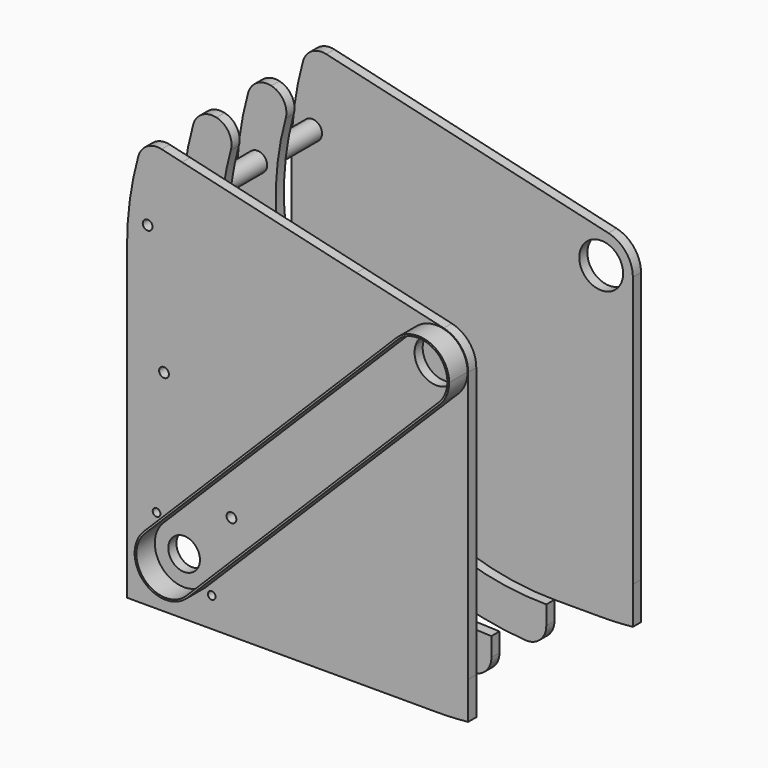
from build123d import *

# Parameters (mm, degrees)
F0_R      = 2.4892
F0_R_2    = 19.1008
F0_R_3    = 3.175
F0_R_4    = 10.31875
F1_DEPTH  = 6.604
F2_R      = 6.35
F2_R_2    = 3.175
F3_DEPTH  = 38.1
F4_R      = 6.35
F4_R_2    = 3.175
F5_DEPTH  = 6.604
F6_R      = 6.35
F6_R_2    = 3.175
F7_DEPTH  = 38.1
F8_R      = 2.15265
F8_R_2    = 6.35
F8_R_3    = 3.175
F9_DEPTH  = 6.604
F10_R     = 6.35
F10_R_2   = 3.175
F10_R_3   = 2.15265
F11_DEPTH = 38.1
F12_R     = 3.175
F12_R_2   = 25.4
F12_R_3   = 14.2875
F12_R_4   = 6.35
F13_DEPTH = 6.604
F14_R     = 12.69999
F16_DEPTH = 15


# Not quite as in the source:
# - a fillet or chamfer is up to 0.001 mm smaller than in the source, because OpenCascade refuses the exact size


with BuildPart() as f1:
    # F0 (on Front) → F1 (new body)
    with BuildSketch(Plane.XZ):
        with BuildLine():
            Line((20.6375, -174.9998249999), (20.6375, -58.3716647869))
            ThreePointArc((20.6375, -58.3716647869), (-43.598353039, -43.9584038442), (-58.5394188118, 20.1567383628))
            Line((-58.5394188118, 20.1567383628), (-166.6121920028, 57.3691784173))
            ThreePointArc((-166.6121920028, 57.3691784173), (-143.4573307784, -102.3271195832), (0, -176.2125))
            ThreePointArc((0, -176.2125), (10.3365490724, -175.9090700036), (20.6375, -174.9998249999))
        make_face()
        with BuildLine():
            ThreePointArc((-92.0202423383, -179.3875), (-172.0465507714, -105.1074903321), (-201.6125, 0))
            Line((-201.6125, 0), (-201.6125, -201.6125))
            Line((-201.6125, -201.6125), (0, -201.6125))
            ThreePointArc((0, -201.6125), (-47.3330635629, -195.9775018975), (-92.0202423383, -179.3875))
        make_face()
        with Locations((-146.444987879, -182.3660123632)):
            Circle(F0_R, mode=Mode.SUBTRACT)
        with Locations((-164.4055001211, -164.4055001211)):
            Circle(F0_R_2, mode=Mode.SUBTRACT)
        with Locations((-182.3660123632, -146.444987879)):
            Circle(F0_R, mode=Mode.SUBTRACT)
        with BuildLine():
            ThreePointArc((0, -176.2125), (-143.4573307784, -102.3271195832), (-166.6121920028, 57.3691784173))
            Line((-166.6121920028, 57.3691784173), (-190.628363823, 65.6386095405))
            ThreePointArc((-190.628363823, 65.6386095405), (-198.8475058399, 33.2756604366), (-201.6125, 0))
            ThreePointArc((-201.6125, 0), (-172.0465507714, -105.1074903321), (-92.0202423383, -179.3875))
            Line((-92.0202423383, -179.3875), (20.6358525902, -179.3875))
            Line((20.6358525902, -179.3875), (20.6358525902, -176.2125))
            Line((20.6358525902, -176.2125), (0, -176.2125))
        make_face()
        with Locations((-133.5813098009, -133.5813098009)):
            Circle(F0_R_3, mode=Mode.SUBTRACT)
        with Locations((-177.5196822242, -64.611880326)):
            Circle(F0_R_3, mode=Mode.SUBTRACT)
        with Locations((-188.1936309033, 16.4648092518)):
            Circle(F0_R_3, mode=Mode.SUBTRACT)
        with BuildLine():
            ThreePointArc((-58.5394188118, 20.1567383628), (-43.598353039, -43.9584038442), (20.6375, -58.3716647869))
            Line((20.6375, -58.3716647869), (20.6375, 0))
            ThreePointArc((20.6375, 0), (-3.4061699659, -20.3544691017), (-19.5131396039, 6.7189127876))
            Line((-19.5131396039, 6.7189127876), (-58.5394188118, 20.1567383628))
        make_face()
        with BuildLine():
            Line((20.6358525902, -179.3875), (-92.0202423383, -179.3875))
            ThreePointArc((-92.0202423383, -179.3875), (-47.3330635629, -195.9775018975), (0, -201.6125))
            ThreePointArc((0, -201.6125), (10.3315003836, -201.347610505), (20.6358525902, -200.5536380725))
            Line((20.6358525902, -200.5536380725), (20.6358525902, -179.3875))
        make_face()
        with BuildLine():
            ThreePointArc((20.6375, 0), (16.1650564357, 12.8295501356), (4.6862116481, 20.0984035843))
            ThreePointArc((4.6862116481, 20.0984035843), (-9.9855967096, 18.0608489447), (-19.5131396039, 6.7189127876))
            ThreePointArc((-19.5131396039, 6.7189127876), (-3.4061699659, -20.3544691017), (20.6375, 0))
        make_face()
        with BuildLine():
            ThreePointArc((19.1008, 0), (-3.15254131, -18.8388440178), (-18.0601612088, 6.2186122047))
            ThreePointArc((-18.0601612088, 6.2186122047), (3.15254131, 18.8388440178), (19.1008, 0))
        make_face(mode=Mode.SUBTRACT)
        with BuildLine():
            ThreePointArc((19.1008, 0), (3.15254131, 18.8388440178), (-18.0601612088, 6.2186122047))
            ThreePointArc((-18.0601612088, 6.2186122047), (-3.15254131, -18.8388440178), (19.1008, 0))
        make_face()
        with BuildLine():
            ThreePointArc((14.2875, 0), (-2.3581176687, -14.091555532), (-13.5090966489, 4.6515550068))
            ThreePointArc((-13.5090966489, 4.6515550068), (2.3581176687, 14.091555532), (14.2875, 0))
        make_face(mode=Mode.SUBTRACT)
        with Locations((-164.4055001211, -164.4055001211)):
            Circle(F0_R_2)
        with Locations((-164.4055001211, -164.4055001211)):
            Circle(F0_R_4, mode=Mode.SUBTRACT)
        with BuildLine():
            ThreePointArc((-58.5394188118, 20.1567383628), (-55.7419247158, 26.9443033911), (-52.1606582139, 33.3530117222))
            Line((-52.1606582139, 33.3530117222), (-165.7422370514, 59.8360761868))
            ThreePointArc((-165.7422370514, 59.8360761868), (-166.1817920957, 58.604241588), (-166.6121920028, 57.3691784173))
            Line((-166.6121920028, 57.3691784173), (-58.5394188118, 20.1567383628))
        make_face()
        with BuildLine():
            Line((4.6862116481, 20.0984035843), (-52.1606582139, 33.3530117222))
            ThreePointArc((-52.1606582139, 33.3530117222), (-55.7419247158, 26.9443033911), (-58.5394188118, 20.1567383628))
            Line((-58.5394188118, 20.1567383628), (-19.5131396039, 6.7189127876))
            ThreePointArc((-19.5131396039, 6.7189127876), (-9.9855967096, 18.0608489447), (4.6862116481, 20.0984035843))
        make_face()
        with BuildLine():
            ThreePointArc((-166.6121920028, 57.3691784173), (-166.1817920957, 58.604241588), (-165.7422370514, 59.8360761868))
            Line((-165.7422370514, 59.8360761868), (-190.628363823, 65.6386095405))
            Line((-190.628363823, 65.6386095405), (-166.6121920028, 57.3691784173))
        make_face()
        with BuildLine():
            Line((20.6375, -176.2125), (20.6375, -174.9998249999))
            ThreePointArc((20.6375, -174.9998249999), (10.3365490724, -175.9090700036), (0, -176.2125))
            Line((0, -176.2125), (20.6358525902, -176.2125))
            Line((20.6358525902, -176.2125), (20.6375, -176.2125))
        make_face()
    extrude(amount=F1_DEPTH)

    # F2 (on face) → F3 (join)
    with BuildSketch(Plane(origin=(0, 0, 0), x_dir=(-1, 0, 0), z_dir=(0, 1, 0))):
        with Locations((188.1936309033, 16.4648092518)):
            Circle(F2_R)
        with Locations((188.1936309033, 16.4648092518)):
            Circle(F2_R_2, mode=Mode.SUBTRACT)
        with Locations((177.5196822242, -64.611880326)):
            Circle(F2_R)
        with Locations((177.5196822242, -64.611880326)):
            Circle(F2_R_2, mode=Mode.SUBTRACT)
        with Locations((133.5813098009, -133.5813098009)):
            Circle(F2_R)
        with Locations((133.5813098009, -133.5813098009)):
            Circle(F2_R_2, mode=Mode.SUBTRACT)
    extrude(amount=F3_DEPTH)

    # F4 (on face) → F5 (join)
    with BuildSketch(Plane(origin=(0, 38.1, 0), x_dir=(-1, 0, 0), z_dir=(0, 1, 0))):
        with BuildLine():
            ThreePointArc((0, -201.6125), (142.561565922, -142.561565922), (201.6125, 0))
            ThreePointArc((201.6125, 0), (198.8475058399, 33.2756604366), (190.628363823, 65.6386095405))
            Line((190.628363823, 65.6386095405), (184.2347646309, 64.1478563629))
            ThreePointArc((184.2347646309, 64.1478563629), (184.9812468491, 62.5077212969), (185.2369380882, 60.7239329891))
            ThreePointArc((185.2369380882, 60.7239329891), (178.5335970044, 54.383771313), (172.5762608982, 61.4295202641))
            Line((172.5762608982, 61.4295202641), (165.7422370514, 59.8360761868))
            ThreePointArc((165.7422370514, 59.8360761868), (173.575198549, 30.3726127442), (176.2125, 0))
            ThreePointArc((176.2125, 0), (124.6010536798, -124.6010536798), (0, -176.2125))
            Line((0, -176.2125), (0, -201.6125))
        make_face()
        with Locations((94.45625, -163.6030240924)):
            Circle(F4_R, mode=Mode.SUBTRACT)
        with Locations((133.5813098009, -133.5813098009)):
            Circle(F4_R, mode=Mode.SUBTRACT)
        with Locations((157.0750031341, -104.9541616453)):
            Circle(F4_R, mode=Mode.SUBTRACT)
        with Locations((177.5196822242, -64.611880326)):
            Circle(F4_R_2, mode=Mode.SUBTRACT)
        with Locations((187.2963273743, -24.6580292878)):
            Circle(F4_R, mode=Mode.SUBTRACT)
        with Locations((188.1936309033, 16.4648092518)):
            Circle(F4_R_2, mode=Mode.SUBTRACT)
        with BuildLine():
            ThreePointArc((185.2369380882, 60.7239329891), (184.9812468491, 62.5077212969), (184.2347646309, 64.1478563629))
            Line((184.2347646309, 64.1478563629), (180.707171605, 63.325350861))
            ThreePointArc((180.707171605, 63.325350861), (181.702951797, 62.1904566991), (182.0619380882, 60.7239329891))
            ThreePointArc((182.0619380882, 60.7239329891), (178.0981628419, 57.6484722739), (176.103853924, 62.252025766))
            Line((176.103853924, 62.252025766), (172.5762608982, 61.4295202641))
            ThreePointArc((172.5762608982, 61.4295202641), (178.5335970044, 54.383771313), (185.2369380882, 60.7239329891))
        make_face()
        with BuildLine():
            ThreePointArc((182.0619380882, 60.7239329891), (181.702951797, 62.1904566991), (180.707171605, 63.325350861))
            Line((180.707171605, 63.325350861), (176.103853924, 62.252025766))
            ThreePointArc((176.103853924, 62.252025766), (178.0981628419, 57.6484722739), (182.0619380882, 60.7239329891))
        make_face()
        with Locations((187.2963273743, -24.6580292878)):
            Circle(F4_R)
        with Locations((187.2963273743, -24.6580292878)):
            Circle(F4_R_2, mode=Mode.SUBTRACT)
        with Locations((157.0750031341, -104.9541616453)):
            Circle(F4_R)
        with Locations((157.0750031341, -104.9541616453)):
            Circle(F4_R_2, mode=Mode.SUBTRACT)
        with Locations((94.45625, -163.6030240924)):
            Circle(F4_R)
        with Locations((187.2963273743, -24.6580292878)):
            Circle(F4_R_2)
        with Locations((157.0750031341, -104.9541616453)):
            Circle(F4_R_2)
        with Locations((133.5813098009, -133.5813098009)):
            Circle(F4_R)
        with Locations((133.5813098009, -133.5813098009)):
            Circle(F4_R_2, mode=Mode.SUBTRACT)
    extrude(amount=F5_DEPTH)

    # F6 (on face) → F7 (join)
    with BuildSketch(Plane(origin=(0, 44.704, 0), x_dir=(-1, 0, 0), z_dir=(0, 1, 0))):
        with Locations((188.1936309033, 16.4648092518)):
            Circle(F6_R)
        with Locations((188.1936309033, 16.4648092518)):
            Circle(F6_R_2, mode=Mode.SUBTRACT)
        with Locations((177.5196822242, -64.611880326)):
            Circle(F6_R)
        with Locations((177.5196822242, -64.611880326)):
            Circle(F6_R_2, mode=Mode.SUBTRACT)
        with Locations((133.5813098009, -133.5813098009)):
            Circle(F6_R)
        with Locations((133.5813098009, -133.5813098009)):
            Circle(F6_R_2, mode=Mode.SUBTRACT)
    extrude(amount=F7_DEPTH)

    # F8 (on face) → F9 (join)
    with BuildSketch(Plane(origin=(0, 82.804, 0), x_dir=(-1, 0, 0), z_dir=(0, 1, 0))):
        with BuildLine():
            ThreePointArc((165.7422370514, 59.8360761868), (144.2128803736, -101.259519506), (0, -176.2125))
            Line((0, -176.2125), (0, -201.6125))
            ThreePointArc((0, -201.6125), (164.1358649446, -117.0769746583), (190.628363823, 65.6386095405))
            Line((190.628363823, 65.6386095405), (178.7684924988, 62.8733218941))
            ThreePointArc((178.7684924988, 62.8733218941), (180.3666221972, 62.2874025156), (181.0395880882, 60.7239329891))
            ThreePointArc((181.0395880882, 60.7239329891), (177.7003055684, 58.9278802935), (178.0425330303, 62.704054733))
            Line((178.0425330303, 62.704054733), (165.7422370514, 59.8360761868))
        make_face()
        with Locations((133.5813098009, -133.5813098009)):
            Circle(F8_R, mode=Mode.SUBTRACT)
        with Locations((157.0750031341, -104.9541616453)):
            Circle(F8_R, mode=Mode.SUBTRACT)
        with Locations((177.5196822242, -64.611880326)):
            Circle(F8_R, mode=Mode.SUBTRACT)
        with Locations((187.2963273743, -24.6580292878)):
            Circle(F8_R, mode=Mode.SUBTRACT)
        with Locations((188.1936309033, 16.4648092518)):
            Circle(F8_R_2, mode=Mode.SUBTRACT)
        with BuildLine():
            Line((178.7684924988, 62.8733218941), (178.0425330303, 62.704054733))
            ThreePointArc((178.0425330303, 62.704054733), (177.7003055684, 58.9278802935), (181.0395880882, 60.7239329891))
            ThreePointArc((181.0395880882, 60.7239329891), (180.3666221972, 62.2874025156), (178.7684924988, 62.8733218941))
        make_face()
        with Locations((157.0750031341, -104.9541616453)):
            Circle(F8_R)
        with Locations((187.2963273743, -24.6580292878)):
            Circle(F8_R)
        with Locations((188.1936309033, 16.4648092518)):
            Circle(F8_R_2)
        with Locations((188.1936309033, 16.4648092518)):
            Circle(F8_R_3, mode=Mode.SUBTRACT)
    extrude(amount=F9_DEPTH)

    # F10 (on face) → F11 (join)
    with BuildSketch(Plane(origin=(0, 89.408, 0), x_dir=(-1, 0, 0), z_dir=(0, 1, 0))):
        with Locations((188.1936309033, 16.4648092518)):
            Circle(F10_R)
        with Locations((188.1936309033, 16.4648092518)):
            Circle(F10_R_2, mode=Mode.SUBTRACT)
        with Locations((177.5196822242, -64.611880326)):
            Circle(F10_R)
        with Locations((177.5196822242, -64.611880326)):
            Circle(F10_R_3, mode=Mode.SUBTRACT)
        with Locations((133.5813098009, -133.5813098009)):
            Circle(F10_R)
        with Locations((133.5813098009, -133.5813098009)):
            Circle(F10_R_3, mode=Mode.SUBTRACT)
    extrude(amount=F11_DEPTH)

    # F12 (on face) → F13 (join)
    with BuildSketch(Plane(origin=(0, 127.508, 0), x_dir=(-1, 0, 0), z_dir=(0, 1, 0))):
        with BuildLine():
            Line((190.628363823, 65.6386095405), (-4.6862116481, 20.0984035843))
            ThreePointArc((-4.6862116481, 20.0984035843), (-16.1650564357, 12.8295501356), (-20.6375, 0))
            Line((-20.6375, 0), (-20.6375, -176.2125))
            Line((-20.6375, -176.2125), (-20.6358525902, -200.5536380725))
            ThreePointArc((-20.6358525902, -200.5536380725), (-10.3315003836, -201.347610505), (0, -201.6125))
            Line((0, -201.6125), (201.6125, -201.6125))
            Line((201.6125, -201.6125), (201.6125, 0))
            ThreePointArc((201.6125, 0), (198.8475058399, 33.2756604366), (190.628363823, 65.6386095405))
        make_face()
        with Locations((133.5813098009, -133.5813098009)):
            Circle(F12_R, mode=Mode.SUBTRACT)
        with Locations((164.4055001211, -164.4055001211)):
            Circle(F12_R_2, mode=Mode.SUBTRACT)
        with Locations((177.5196822242, -64.611880326)):
            Circle(F12_R, mode=Mode.SUBTRACT)
        Circle(F12_R_3, mode=Mode.SUBTRACT)
        with Locations((188.1936309033, 16.4648092518)):
            Circle(F12_R_4, mode=Mode.SUBTRACT)
        with Locations((188.1936309033, 16.4648092518)):
            Circle(F12_R_4)
        with Locations((188.1936309033, 16.4648092518)):
            Circle(F12_R, mode=Mode.SUBTRACT)
    extrude(amount=F13_DEPTH)

    # F14 (radius 12.7 in the source; OpenCascade refuses exactly that, so slightly less here)
    f14_edges = [f1.edges().sort_by_distance(p)[0] for p in [
        (-190.628364, -3.302, 65.63861),
        (-190.628364, 41.402, 65.63861),
        (-165.742237, 86.106, 59.836076),
        (-190.628364, 86.106, 65.63861),
        (-165.742237, 41.402, 59.836076),
        (-190.628364, 130.81, 65.63861),
        (0, 41.402, -201.6125),
        (0, 86.106, -201.6125),
    ]]
    fillet(f14_edges, radius=F14_R)


with BuildPart() as f16:
    # F15 (on face) → F16 (new body)
    with BuildSketch(Plane.XZ.offset(6.604)):
        with BuildLine():
            ThreePointArc((-14.314528257, 12.6465347594), (6.7609769749, 17.8642030605), (19.1008, 0))
            ThreePointArc((19.1008, 0), (17.4126317909, -7.8511664582), (12.6465347594, -14.314528257))
            Line((12.6465347594, -14.314528257), (8.6658675036, -18.2951955128))
            ThreePointArc((8.6658675036, -18.2951955128), (11.6613067569, -16.5476694178), (14.314528257, -14.314528257))
            ThreePointArc((14.314528257, -14.314528257), (18.7028324803, -7.7469668681), (20.2438, 0))
            ThreePointArc((20.2438, 0), (7.7469668681, 18.7028324803), (-14.314528257, 14.314528257))
            ThreePointArc((-14.314528257, 14.314528257), (-16.5476694178, 11.6613067569), (-18.2951955128, 8.6658675036))
            Line((-18.2951955128, 8.6658675036), (-14.314528257, 12.6465347594))
        make_face()
        with BuildLine():
            Line((-173.0713676247, -146.1103046083), (-18.2951955128, 8.6658675036))
            ThreePointArc((-18.2951955128, 8.6658675036), (-16.5476694178, 11.6613067569), (-14.314528257, 14.314528257))
            Line((-14.314528257, 14.314528257), (-178.7200283781, -150.0909718641))
            ThreePointArc((-178.7200283781, -150.0909718641), (-176.066806878, -147.8578307033), (-173.0713676247, -146.1103046083))
        make_face()
        with BuildLine():
            ThreePointArc((14.314528257, -14.314528257), (11.6613067569, -16.5476694178), (8.6658675036, -18.2951955128))
            Line((8.6658675036, -18.2951955128), (-146.1103046083, -173.0713676247))
            ThreePointArc((-146.1103046083, -173.0713676247), (-147.8578307033, -176.066806878), (-150.0909718641, -178.7200283781))
            Line((-150.0909718641, -178.7200283781), (14.314528257, -14.314528257))
        make_face()
        with BuildLine():
            Line((-177.0520348805, -150.0909718641), (-173.0713676247, -146.1103046083))
            ThreePointArc((-173.0713676247, -146.1103046083), (-176.066806878, -147.8578307033), (-178.7200283781, -150.0909718641))
            ThreePointArc((-178.7200283781, -150.0909718641), (-178.7200283781, -178.7200283781), (-150.0909718641, -178.7200283781))
            ThreePointArc((-150.0909718641, -178.7200283781), (-147.8578307033, -176.066806878), (-146.1103046083, -173.0713676247))
            Line((-146.1103046083, -173.0713676247), (-150.0909718641, -177.0520348805))
            ThreePointArc((-150.0909718641, -177.0520348805), (-177.9118053272, -177.9118053272), (-177.0520348805, -150.0909718641))
        make_face()
    extrude(amount=F16_DEPTH)


solid = Compound([f1.part, f16.part])
